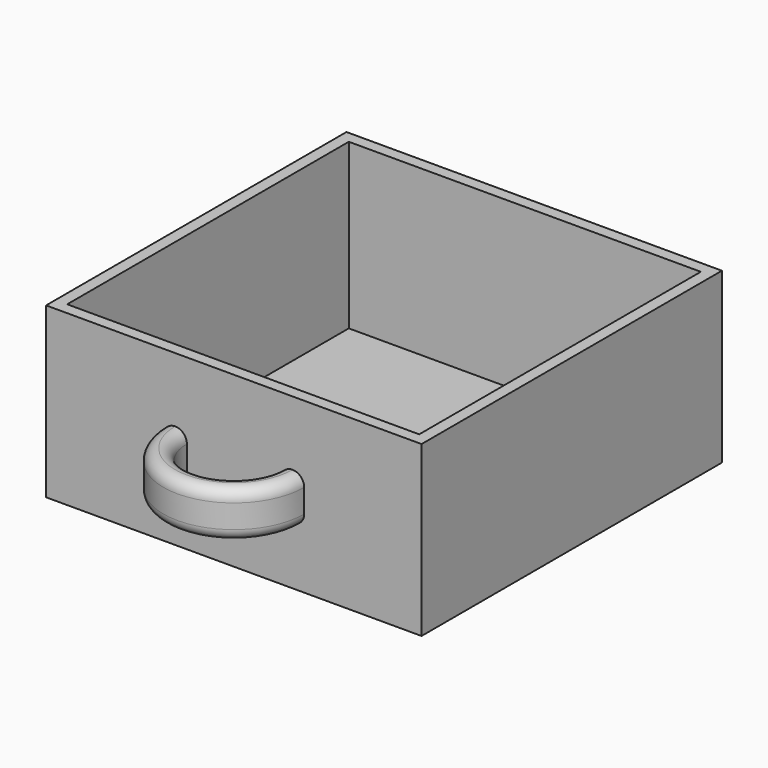
from build123d import *

# Parameters (mm, degrees)
F0_W     = 101.6
F0_H     = 45.72
F1_DEPTH = 101.6
F2_W     = 95.25
F2_H     = 95.25
F3_DEPTH = 44.45
F4_W     = 19.05
F4_H     = 6.35
F5_ANGLE = 180
F7_DEPTH = 25.4
F8_R     = 3.17499


# Not quite as in the source:
# - a fillet or chamfer is up to 0.001 mm smaller than in the source, because OpenCascade refuses the exact size


with BuildPart() as f1:
    # F0 (on Front) → F1 (new body)
    with BuildSketch(Plane.XZ):
        with Locations((17.3888143581, 4.6649015626)):
            Rectangle(F0_W, F0_H)
    extrude(amount=-F1_DEPTH)

    # F2 (on face) → F3 (cut)
    with BuildSketch(Plane.XY.offset(27.5249015626)):
        with Locations((17.3888143581, 50.8)):
            Rectangle(F2_W, F2_H)
    extrude(amount=-F3_DEPTH, mode=Mode.SUBTRACT)

    # F4 (on face) → F5 (revolve)
    with BuildSketch(Plane.XZ):
        with Locations((7.8638143581, 6.8874015626)):
            Rectangle(F4_W, F4_H)
        with Locations((7.8638143581, 0.5374015626)):
            Rectangle(F4_W, F4_H)
    revolve(axis=Axis((17.3888143581, 0, 3.7124015626), (0, 0, 1)), revolution_arc=F5_ANGLE)

    # F6 (on face) → F7 (cut)
    with BuildSketch(Plane.XY.offset(10.0624015626)):
        with BuildLine():
            Line((30.0888143581, 0), (4.6888143581, 0))
            ThreePointArc((4.6888143581, 0), (17.3888143581, -12.7), (30.0888143581, 0))
        make_face()
    extrude(amount=-F7_DEPTH, mode=Mode.SUBTRACT)

    # F8 (radius 3.175 in the source; OpenCascade refuses exactly that, so slightly less here)
    f8_edges = [f1.edges().sort_by_distance(p)[0] for p in [
        (17.388814, -19.05, 10.062402),
        (17.388814, -12.7, 10.062402),
        (17.388814, -19.05, -2.637598),
        (17.388814, -12.7, -2.637598),
    ]]
    fillet(f8_edges, radius=F8_R)


solid = f1.part
